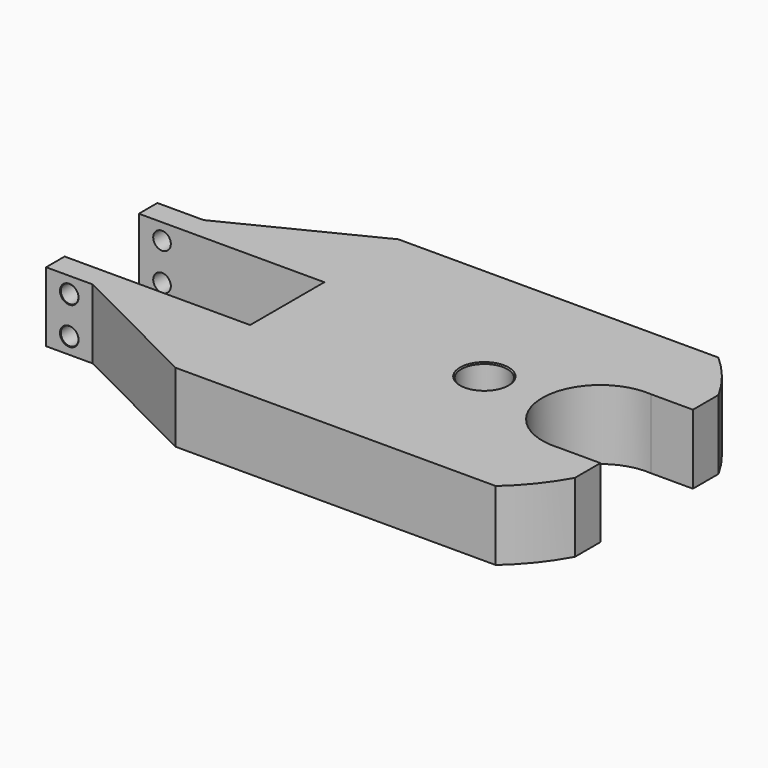
from build123d import *

# Parameters (mm, degrees)
F1_DEPTH = 38.1


# Not quite as in the source:
# - a pattern or mirror of a feature is missing from the dataset's text; its kind, count and spacing are read off the source's solid


with BuildPart() as f1:
    # F0 (on Top) → F1 (new body)
    with BuildSketch(Plane.XY):
        with BuildLine():
            Line((0, 25.4), (0, 0))
            Line((0, 0), (0, -25.4))
            Line((0, -25.4), (-101.6, -25.4))
            Line((-101.6, -25.4), (-101.6, -38.1))
            Line((-101.6, -38.1), (-76.2, -38.1))
            Line((-76.2, -38.1), (-0.1165057322, -76.2))
            Line((-0.1165057322, -76.2), (175.152083301, -76.2))
            ThreePointArc((175.152083301, -76.2), (187.161060787, -63.6252139407), (196.85, -49.1868884968))
            Line((196.85, -49.1868884968), (196.85, -31.6608884968))
            Line((196.85, -31.6608884968), (173.8271074, -31.6608884968))
            ThreePointArc((173.8271074, -31.6608884968), (139.7, 0), (173.8271074, 31.6608884968))
            Line((173.8271074, 31.6608884968), (196.85, 31.6608884968))
            Line((196.85, 31.6608884968), (196.85, 49.1868884968))
            ThreePointArc((196.85, 49.1868884968), (187.161060787, 63.6252139407), (175.152083301, 76.2))
            Line((175.152083301, 76.2), (-0.1165057322, 76.2))
            Line((-0.1165057322, 76.2), (-76.2, 38.1))
            Line((-76.2, 38.1), (-101.6, 38.1))
            Line((-101.6, 38.1), (-101.6, 25.4))
            Line((-101.6, 25.4), (0, 25.4))
        make_face()
    extrude(amount=F1_DEPTH)

    # F3 (on offset) → F4 (revolve, cut)
    with BuildSketch(Plane(origin=(107.95, 0, 0), x_dir=(0, -1, 0), z_dir=(-1, 0, 0))):
        Polygon((-13.335, 0), (0, 0), (0, 38.1), (-13.335, 38.1), (-12.7, 37.465), (-12.7, 0.635), align=None)
    revolve(axis=Axis((107.95, 0, 19.05), (0, 0, 1)), mode=Mode.SUBTRACT)

    # F6 (on mid) → F7 (revolve, cut)
    with BuildSketch(Plane.XY.offset(19.05)):
        Polygon((24.7731973962, 0), (0, 0), (0, -10.16), (0.635, -9.525), (19.05, -9.525), align=None)
    revolve(axis=Axis((12.3865986981, 0, 19.05), (1, 0, 0)), mode=Mode.SUBTRACT)

    # F9 (on offset) → F10 (revolve, cut)
    with BuildSketch(Plane(origin=(-88.9, 0, 0), x_dir=(0, -1, 0), z_dir=(-1, 0, 0))):
        Polygon((38.1, 8.89), (-38.1, 8.89), (-38.1, 3.81), (-37.846, 4.064), (37.846, 4.064), (38.1, 3.81), align=None)
    f10 = revolve(axis=Axis((-88.9, 0, 8.89), (0, 1, 0)), mode=Mode.SUBTRACT)

    # F10_copies: F10 across plane
    add(f10.mirror(Plane.XY.offset(19.05)), mode=Mode.SUBTRACT)


solid = f1.part
